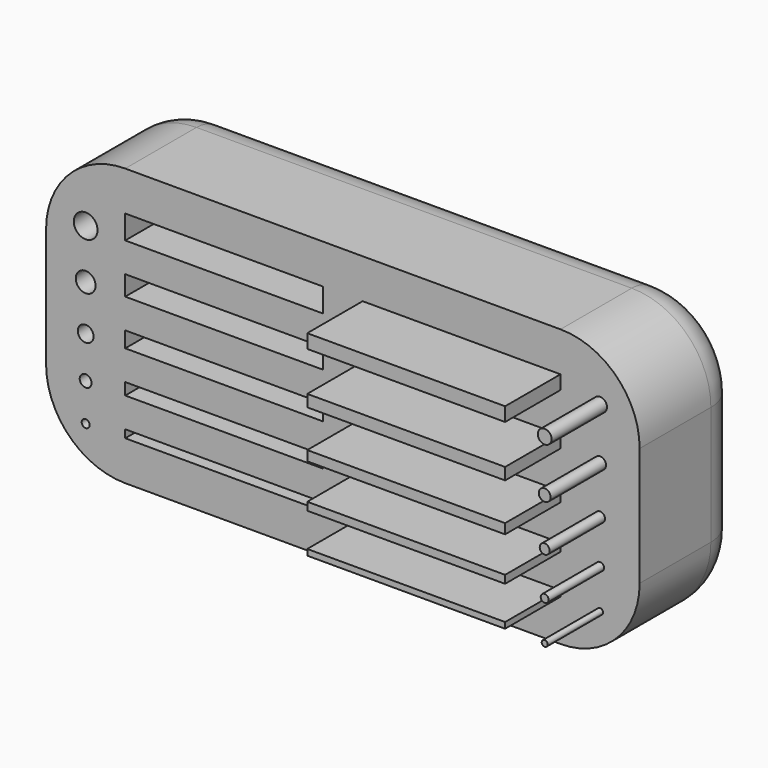
from build123d import *

# Parameters (mm, degrees)
F0_W         = 30
F0_H         = 14
F0_R         = 0.2
F0_W_2       = 10
F0_H_2       = 0.4
F0_R_2       = 0.3
F0_R_3       = 0.4
F0_H_3       = 0.6
F0_H_4       = 0.8
F0_H_5       = 0.3
F0_R_4       = 0.15
F0_H_6       = 0.5
F0_R_5       = 0.25
F0_R_6       = 0.5
F0_H_7       = 1
F0_R_7       = 0.6
F0_H_8       = 1.2
F0_H_9       = 0.7
F0_R_8       = 0.35
F1_DEPTH     = 6.5
F2_DEPTH     = 3.5
F3_W         = 30
F3_H         = 14
F4_DEPTH     = 1
F5_R         = 2
F6_T1_DEPTH  = 16.5
F6_T4_ANGLE  = 90
F6_T6_ANGLE  = 90
F6_T8_ANGLE  = 90
F6_T10_ANGLE = 90


# Not quite as in the source:
# - a fillet or chamfer that OpenCascade refuses, or shapes differently, is made with other operations: its cross-section is extruded or revolved along the edge and cut away or added


with BuildPart() as f1:
    # F0 (on Front) → F1 (new body)
    with BuildSketch(Plane.XZ):
        with Locations((11, -5)):
            Rectangle(F0_W, F0_H)
        with Locations((-2, -10)):
            Circle(F0_R, mode=Mode.SUBTRACT)
        with Locations((5, -9.8)):
            Rectangle(F0_W_2, F0_H_2, mode=Mode.SUBTRACT)
        with Locations((-2, -8.1)):
            Circle(F0_R_2, mode=Mode.SUBTRACT)
        with Locations((-2, -6)):
            Circle(F0_R_3, mode=Mode.SUBTRACT)
        with Locations((5, -7.8)):
            Rectangle(F0_W_2, F0_H_3, mode=Mode.SUBTRACT)
        with Locations((5, -5.6)):
            Rectangle(F0_W_2, F0_H_4, mode=Mode.SUBTRACT)
        with Locations((17, -9.75)):
            Rectangle(F0_W_2, F0_H_5, mode=Mode.SUBTRACT)
        with Locations((24, -9.9)):
            Circle(F0_R_4, mode=Mode.SUBTRACT)
        with Locations((17, -7.7)):
            Rectangle(F0_W_2, F0_H_2, mode=Mode.SUBTRACT)
        with Locations((17, -5.45)):
            Rectangle(F0_W_2, F0_H_6, mode=Mode.SUBTRACT)
        with Locations((24, -7.9)):
            Circle(F0_R, mode=Mode.SUBTRACT)
        with Locations((24, -5.7)):
            Circle(F0_R_5, mode=Mode.SUBTRACT)
        with Locations((-2, -3.7)):
            Circle(F0_R_6, mode=Mode.SUBTRACT)
        with Locations((5, -3.2)):
            Rectangle(F0_W_2, F0_H_7, mode=Mode.SUBTRACT)
        with Locations((-2, -1.2)):
            Circle(F0_R_7, mode=Mode.SUBTRACT)
        with Locations((5, -0.6)):
            Rectangle(F0_W_2, F0_H_8, mode=Mode.SUBTRACT)
        with Locations((17, -3)):
            Rectangle(F0_W_2, F0_H_3, mode=Mode.SUBTRACT)
        with Locations((24, -3.3)):
            Circle(F0_R_2, mode=Mode.SUBTRACT)
        with Locations((17, -0.35)):
            Rectangle(F0_W_2, F0_H_9, mode=Mode.SUBTRACT)
        with Locations((24, -0.7)):
            Circle(F0_R_8, mode=Mode.SUBTRACT)
        with Locations((17, -0.35)):
            Rectangle(F0_W_2, F0_H_9)
        with Locations((17, -3)):
            Rectangle(F0_W_2, F0_H_3)
        with Locations((17, -5.45)):
            Rectangle(F0_W_2, F0_H_6)
        with Locations((17, -7.7)):
            Rectangle(F0_W_2, F0_H_2)
        with Locations((17, -9.75)):
            Rectangle(F0_W_2, F0_H_5)
        with Locations((24, -0.7)):
            Circle(F0_R_8)
        with Locations((24, -3.3)):
            Circle(F0_R_2)
        with Locations((24, -5.7)):
            Circle(F0_R_5)
        with Locations((24, -7.9)):
            Circle(F0_R)
        with Locations((24, -9.9)):
            Circle(F0_R_4)
    extrude(amount=-F1_DEPTH)

    # F0 (on Front) → F2 (join)
    with BuildSketch(Plane.XZ):
        with Locations((17, -0.35)):
            Rectangle(F0_W_2, F0_H_9)
        with Locations((17, -3)):
            Rectangle(F0_W_2, F0_H_3)
        with Locations((17, -5.45)):
            Rectangle(F0_W_2, F0_H_6)
        with Locations((17, -7.7)):
            Rectangle(F0_W_2, F0_H_2)
        with Locations((17, -9.75)):
            Rectangle(F0_W_2, F0_H_5)
        with Locations((24, -0.7)):
            Circle(F0_R_8)
        with Locations((24, -3.3)):
            Circle(F0_R_2)
        with Locations((24, -5.7)):
            Circle(F0_R_5)
        with Locations((24, -7.9)):
            Circle(F0_R)
        with Locations((24, -9.9)):
            Circle(F0_R_4)
    extrude(amount=F2_DEPTH)

    # F3 (on face) → F4 (join)
    with BuildSketch(Plane(origin=(0, 6.5, 0), x_dir=(-1, 0, 0), z_dir=(0, 1, 0))):
        with Locations((-11, -5)):
            Rectangle(F3_W, F3_H)
    extrude(amount=-F4_DEPTH)

    # F5
    f5_edges = [f1.edges().sort_by_distance(p)[0] for p in [
        (-4, 6.5, -5),
        (11, 6.5, -12),
        (26, 6.5, -5),
        (11, 6.5, 2),
    ]]
    fillet(f5_edges, radius=F5_R)

    # F6: fillet of radius 4 on 4 edges, made by hand

    # F6_s2 → F6_t1 (cut)
    with BuildSketch(Plane.XZ.offset(-6.5)):
        with BuildLine():
            ThreePointArc((-4, -8), (-2.8284271247, -10.8284271247), (0, -12))
            Line((0, -12), (-4, -12))
            Line((-4, -12), (-4, -8))
        make_face()
        with BuildLine():
            ThreePointArc((0, 2), (-2.8284271247, 0.8284271247), (-4, -2))
            Line((-4, -2), (-4, 2))
            Line((-4, 2), (0, 2))
        make_face()
        with BuildLine():
            ThreePointArc((26, -8), (24.8284271247, -10.8284271247), (22, -12))
            Line((22, -12), (26, -12))
            Line((26, -12), (26, -8))
        make_face()
        with BuildLine():
            ThreePointArc((22, 2), (24.8284271247, 0.8284271247), (26, -2))
            Line((26, -2), (26, 2))
            Line((26, 2), (22, 2))
        make_face()
    extrude(amount=F6_T1_DEPTH, mode=Mode.SUBTRACT)

    # F6_s3 → F6_t4 (revolve, cut)
    with BuildSketch(Plane.YZ.offset(22)):
        with BuildLine():
            ThreePointArc((6.5, 0), (5.9142135624, 1.4142135624), (4.5, 2))
            Line((4.5, 2), (6.5, 2))
            Line((6.5, 2), (6.5, 0))
        make_face()
    revolve(axis=Axis((22, 6.5, -2), (0, 1, 0)), revolution_arc=F6_T4_ANGLE, mode=Mode.SUBTRACT)

    # F6_s5 → F6_t6 (revolve, cut)
    with BuildSketch(Plane.XY.offset(-8)):
        with BuildLine():
            ThreePointArc((24, 6.5), (25.4142135624, 5.9142135624), (26, 4.5))
            Line((26, 4.5), (26, 6.5))
            Line((26, 6.5), (24, 6.5))
        make_face()
    revolve(axis=Axis((22, 6.5, -8), (0, 1, 0)), revolution_arc=F6_T6_ANGLE, mode=Mode.SUBTRACT)

    # F6_s7 → F6_t8 (revolve, cut)
    with BuildSketch(Plane.XY.offset(-2)):
        with BuildLine():
            ThreePointArc((-2, 6.5), (-3.4142135624, 5.9142135624), (-4, 4.5))
            Line((-4, 4.5), (-4, 6.5))
            Line((-4, 6.5), (-2, 6.5))
        make_face()
    revolve(axis=Axis((0, 6.5, -2), (0, 1, 0)), revolution_arc=F6_T8_ANGLE, mode=Mode.SUBTRACT)

    # F6_s9 → F6_t10 (revolve, cut)
    with BuildSketch(Plane.YZ):
        with BuildLine():
            ThreePointArc((6.5, -10), (5.9142135624, -11.4142135624), (4.5, -12))
            Line((4.5, -12), (6.5, -12))
            Line((6.5, -12), (6.5, -10))
        make_face()
    revolve(axis=Axis((0, 6.5, -8), (0, 1, 0)), revolution_arc=F6_T10_ANGLE, mode=Mode.SUBTRACT)


solid = f1.part
